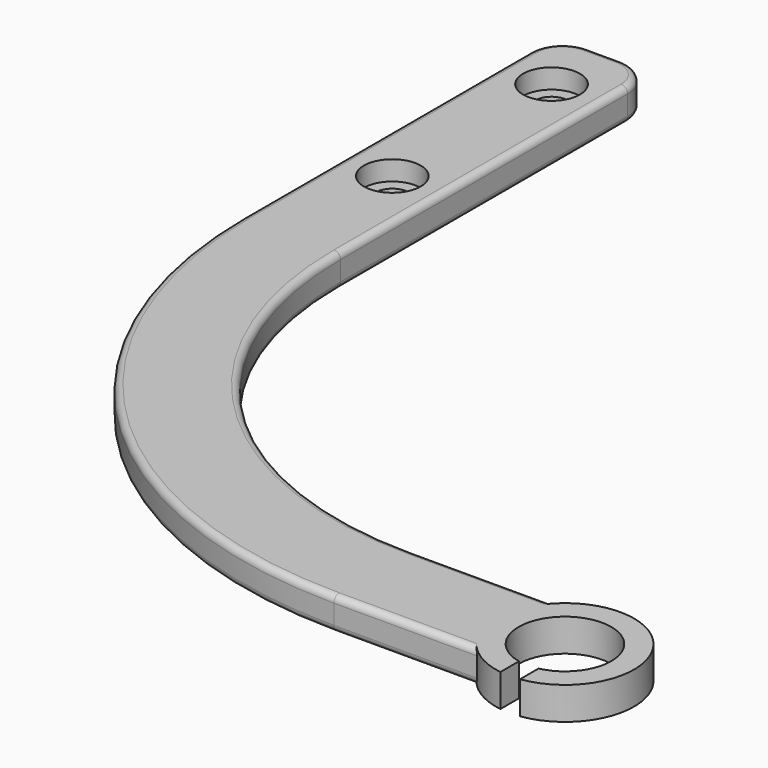
from build123d import *

# Parameters (mm, degrees)
F0_R     = 2.5
F1_DEPTH = 5
F3_R     = 4.35
F4_DEPTH = 3
F5_R     = 5
F6_R     = 5
F7_R     = 1
F8_R     = 1


# Not quite as in the source:
# - a feature names something its author has since deleted; it is built from what else it names


with BuildPart() as f1:
    # F0 (on Top) → F1 (new body)
    with BuildSketch(Plane.XY):
        with BuildLine():
            Line((148.606140697, -2.9933312156), (148.606140697, 0.5602593708))
            ThreePointArc((148.606140697, 0.5602593708), (150.106140697, 14.6), (151.606140697, 0.5602593708))
            Line((151.606140697, 0.5602593708), (151.606140697, -2.9933312156))
            ThreePointArc((151.606140697, -2.9933312156), (159.5883343472, 12.2379324162), (142.615479845, 15))
            Line((142.615479845, 15), (120.706140697, 15))
            ThreePointArc((120.706140697, 15), (81.8152677317, 31.1091270347), (65.706140697, 70))
            Line((65.706140697, 70), (65.706140697, 130))
            Line((65.706140697, 130), (50.706140697, 130))
            Line((50.706140697, 130), (50.706140697, 70))
            ThreePointArc((50.706140697, 70), (71.2086660139, 20.5025253169), (120.706140697, 0))
            Line((120.706140697, 0), (142.615479845, 0))
            ThreePointArc((142.615479845, 0), (145.3682082808, -1.9821936502), (148.606140697, -2.9933312156))
        make_face()
        with Locations((58.206140697, 89.3)):
            Circle(F0_R, mode=Mode.SUBTRACT)
        with Locations((58.206140697, 119.8)):
            Circle(F0_R, mode=Mode.SUBTRACT)
    extrude(amount=F1_DEPTH)

    # F3 (on offset) → F4 (cut, through all)
    with BuildSketch(Plane.XY.offset(2)):
        with Locations((58.206140697, 119.8)):
            Circle(F3_R)
        with Locations((58.206140697, 89.3)):
            Circle(F3_R)
    extrude(amount=F4_DEPTH, mode=Mode.SUBTRACT)

    # F5
    f5_edges = [f1.edges().sort_by_distance(p)[0] for p in [
        (50.706141, 130, 2.5),
    ]]
    fillet(f5_edges, radius=F5_R)

    # F6
    f6_edges = [f1.edges().sort_by_distance(p)[0] for p in [
        (65.706141, 130, 2.5),
    ]]
    fillet(f6_edges, radius=F6_R)

    # F7
    f7_edges = [f1.edges().sort_by_distance(p)[0] for p in [
        (50.706141, 97.5, 5),
    ]]
    fillet(f7_edges, radius=F7_R)

    # F8
    f8_edges = [f1.edges().sort_by_distance(p)[0] for p in [
        (50.706141, 97.5, 0),
    ]]
    fillet(f8_edges, radius=F8_R)


solid = f1.part
